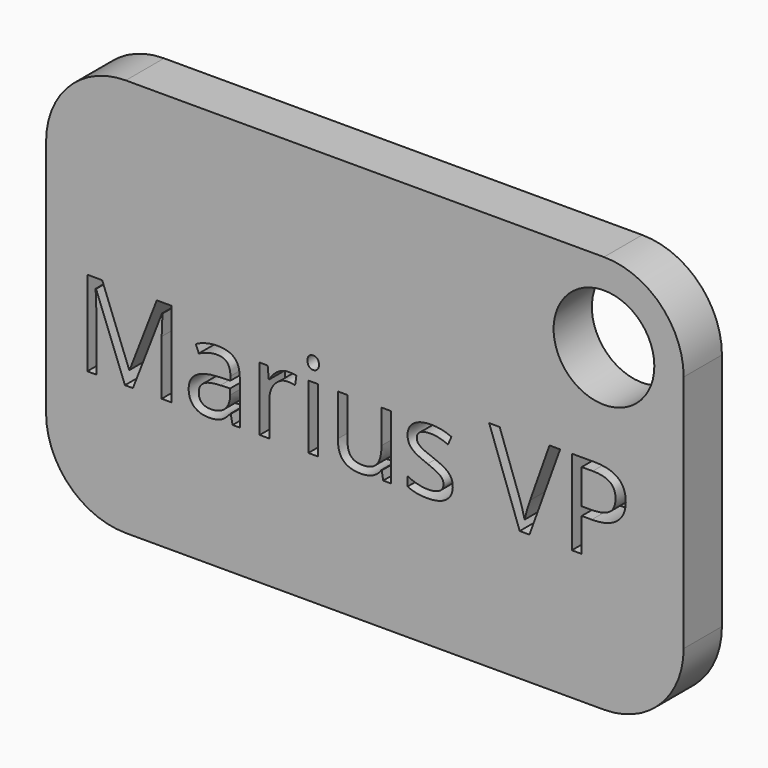
from build123d import *

# Parameters (mm, degrees)
F1_DEPTH     = 3
F2_R         = 3.1596060778
F3_DEPTH     = 3
F4_TEXT_SIZE = 7.4761364395
F5_DEPTH     = 2


# Not quite as in the source:
# - Text() gives the source's letters only with a copy of the font that has no kerning and outlines rounded to 1/6400 em; it was checked with that copy


with BuildPart() as f1:
    # F0 (on Front) → F1 (new body)
    with BuildSketch(Plane.XZ):
        with BuildLine():
            ThreePointArc((0, 5), (1.4644660941, 1.4644660941), (5, 0))
            Line((5, 0), (35, 0))
            ThreePointArc((35, 0), (38.5355339059, 1.4644660941), (40, 5))
            Line((40, 5), (40, 20))
            ThreePointArc((40, 20), (38.5355339059, 23.5355339059), (35, 25))
            Line((35, 25), (5, 25))
            ThreePointArc((5, 25), (1.4644660941, 23.5355339059), (0, 20))
            Line((0, 20), (0, 5))
        make_face()
    extrude(amount=F1_DEPTH)

    # F2 (on face) → F3 (cut)
    with BuildSketch(Plane.XZ.offset(3)):
        with Locations((35, 20)):
            Circle(F2_R)
    extrude(amount=-F3_DEPTH, mode=Mode.SUBTRACT)

    # F4 (on face) → F5 (cut)
    with BuildSketch(Plane.XZ.offset(3)):
        with Locations((1.8519152877, 8.1482900945)):
            Text('Marius VP', F4_TEXT_SIZE, font='Open Sans', text_align=(TextAlign.LEFT, TextAlign.BOTTOM))
    extrude(amount=-F5_DEPTH, mode=Mode.SUBTRACT)


solid = f1.part
